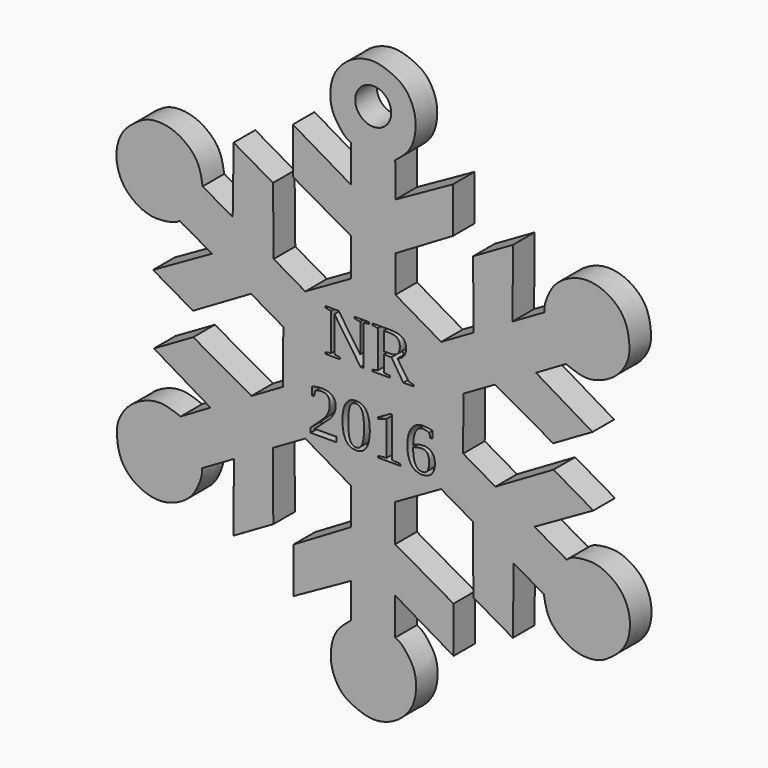
from build123d import *

# Parameters (mm, degrees)
F1_DEPTH     = 3
F3_D         = 4
F4_TEXT_SIZE = 7.1690029775
F5_DEPTH     = 1.5


# Not quite as in the source:
# - Text() gives the source's letters only with a copy of the font that has no kerning and outlines rounded to 1/6400 em; it was checked with that copy


with BuildPart() as f1:
    # F0 (on Front) → F1 (new body)
    with BuildSketch(Plane.XZ):
        with BuildLine():
            add(Edge.make_bspline(
                [(37.2373796999, 9.4348983839), (37.4251641018, 9.3510028964), (37.8701899406, 9.1521809532), (38.6817217589, 8.1752111907), (39.4062988326, 7.0113605624), (39.6519953422, 5.3867909556), (39.3224060532, 3.2517367706), (37.6206347845, 1.2780817822), (35.0148704912, 0.371790515), (32.7778145975, 1.1156204474), (31.2129824114, 1.9875750422), (30.1474541561, 3.8790702997), (29.9862610461, 5.8902465417), (30.532836937, 8.0610699246), (31.7339680071, 9.036908188), (32.3466956615, 9.5347082242)],
                knots=[0, 0, 0, 0, 0.0459998317, 0.1090139196, 0.1754280111, 0.246904677, 0.3288017158, 0.4185892321, 0.5104257569, 0.5955487448, 0.6705198642, 0.7515537915, 0.8317987285, 0.9141962329, 1, 1, 1, 1], degree=3))
            Line((37.2373796999, 9.4348983839), (37.2373796999, 13.5579572657))
            Line((37.2373796999, 13.5579572657), (43.718758629, 9.7468400041))
            Line((43.718758629, 9.7468400041), (43.718758629, 14.8636193613))
            Line((43.718758629, 14.8636193613), (37.2373796999, 18.5688713232))
            Line((37.2373796999, 18.5688713232), (37.2373796999, 22.7115825247))
            Line((37.2373796999, 22.7115825247), (42.3384769651, 25.6261969935))
            Line((42.3384769651, 25.6261969935), (45.8529271634, 23.5971282255))
            Line((45.8529271634, 23.5971282255), (45.9293157475, 16.177781961))
            Line((45.9293157475, 16.177781961), (50.2994563725, 13.6546800947))
            Line((50.2994563725, 13.6546800947), (50.40642864, 20.9681629222))
            Line((50.40642864, 20.9681629222), (53.7508636268, 19.0672780077))
            add(Edge.make_bspline(
                [(56.2826435033, 23.2528297066), (56.4533267724, 23.3765045131), (56.839458541, 23.7361558524), (58.1039257682, 23.9168971573), (59.4727716087, 23.9733834526), (61.002950547, 23.3705901097), (62.6870351656, 22.0186766462), (63.5454277802, 19.5577567309), (63.0273958428, 16.8480186494), (61.264728006, 15.2826441221), (59.7270664918, 14.363176773), (57.556649242, 14.3871852923), (55.7326931115, 15.2492433393), (54.1380932906, 16.8175392077), (53.8742690919, 18.2961027509), (53.7508636268, 19.0672780077)],
                knots=[0, 0, 0, 0, 0.0471420247, 0.110140019, 0.1765371486, 0.2479955595, 0.329871682, 0.4196362669, 0.5114493369, 0.5965505847, 0.6715025566, 0.7525157881, 0.8327402308, 0.9151166911, 1, 1, 1, 1], degree=3))
            Line((56.2826435033, 23.2528297066), (52.7119697703, 25.3143591476))
            Line((52.7119697703, 25.3143591476), (59.2531836002, 29.0218393209))
            Line((59.2531836002, 29.0218393209), (54.8219226914, 31.5802289995))
            Line((54.8219226914, 31.5802289995), (48.3723909003, 27.8198161763))
            Line((48.3723909003, 27.8198161763), (44.7846977593, 29.891171777))
            Line((44.7846977593, 29.891171777), (44.8111162197, 35.7661588302))
            Line((44.8111162197, 35.7661588302), (48.325566418, 37.7952275983))
            Line((48.325566418, 37.7952275983), (54.7891030546, 34.1517089204))
            Line((54.7891030546, 34.1517089204), (59.1592436796, 36.6748107867))
            Line((59.1592436796, 36.6748107867), (52.8790678946, 40.4241929016))
            Line((52.8790678946, 40.4241929016), (56.1975000137, 42.3701161042))
            add(Edge.make_bspline(
                [(53.8385958517, 46.6554776435), (53.8178644494, 46.8551850525), (53.7788826284, 47.3092452721), (54.2124163427, 48.5077384287), (54.8592955807, 49.7124607744), (56.1429910302, 50.7389428582), (58.1569163578, 51.5205869261), (60.7170003528, 51.0337692557), (62.8047652541, 49.2302436061), (63.2791107249, 46.920905952), (63.3064071223, 45.1300249509), (62.2010312841, 43.2603978107), (60.5401138614, 42.1194060959), (58.3836859108, 41.4904279159), (56.9379088943, 42.0872561597), (56.1975000137, 42.3701161042)],
                knots=[0, 0, 0, 0, 0.0449055887, 0.1079742905, 0.1744459427, 0.2459845569, 0.3279525753, 0.4178179099, 0.5097340288, 0.5949307923, 0.6699668886, 0.7510710474, 0.8313855322, 0.91385445, 1, 1, 1, 1], degree=3))
            Line((53.8385958517, 46.6554776435), (50.2679221188, 44.5939482026))
            Line((50.2679221188, 44.5939482026), (50.3277570196, 52.1125456375))
            Line((50.3277570196, 52.1125456375), (45.8964961107, 49.5541559589))
            Line((45.8964961107, 49.5541559589), (45.9283432488, 42.0884911738))
            Line((45.9283432488, 42.0884911738), (42.3406501078, 40.0171355731))
            Line((42.3406501078, 40.0171355731), (37.265971303, 42.9775081575))
            Line((37.265971303, 42.9775081575), (37.265971303, 47.0356456935))
            Line((37.265971303, 47.0356456935), (43.6531193554, 50.8114732802))
            Line((43.6531193554, 50.8114732802), (43.6531193554, 55.8576770127))
            Line((43.6531193554, 55.8576770127), (37.265971303, 52.2935763001))
            Line((37.265971303, 52.2935763001), (37.2399684352, 56.1403844172))
            add(Edge.make_bspline(
                [(32.3492843968, 56.2401942576), (32.1614999949, 56.3240897451), (31.7164741562, 56.5229116883), (30.9049423379, 57.4998814507), (30.1803652642, 58.6637320791), (29.9346687546, 60.2883016859), (30.2642580436, 62.4233558709), (31.9660293123, 64.3970108593), (34.5717936056, 65.3033021265), (36.8088494992, 64.5594721941), (38.3736816853, 63.6875175993), (39.4392099407, 61.7960223418), (39.6004030507, 59.7848460998), (39.0538271598, 57.6140227169), (37.8526960896, 56.6381844535), (37.2399684352, 56.1403844172)],
                knots=[0, 0, 0, 0, 0.0459998317, 0.1090139196, 0.1754280111, 0.246904677, 0.3288017158, 0.4185892321, 0.5104257569, 0.5955487448, 0.6705198642, 0.7515537915, 0.8317987285, 0.9141962329, 1, 1, 1, 1], degree=3))
            Line((32.3492843968, 56.2401942576), (32.3492843968, 52.1171353757))
            Line((32.3492843968, 52.1171353757), (25.8679054677, 55.9282526374))
            Line((25.8679054677, 55.9282526374), (25.8679054677, 50.8114732802))
            Line((25.8679054677, 50.8114732802), (32.3492843968, 47.1062213182))
            Line((32.3492843968, 47.1062213182), (32.3492843968, 42.9635101168))
            Line((32.3492843968, 42.9635101168), (27.2481871317, 40.048895648))
            Line((27.2481871317, 40.048895648), (23.7337369334, 42.077964416))
            Line((23.7337369334, 42.077964416), (23.6573483493, 49.4973106805))
            Line((23.6573483493, 49.4973106805), (19.2872077243, 52.0204125467))
            Line((19.2872077243, 52.0204125467), (19.1802354567, 44.7069297193))
            Line((19.1802354567, 44.7069297193), (15.83580047, 46.6078146338))
            add(Edge.make_bspline(
                [(13.3040205935, 42.4222629348), (13.1374508396, 42.3015687263), (12.7316317675, 42.0337442948), (11.4853994243, 41.8099865936), (10.1133856971, 41.7673638515), (8.5841616668, 42.3659788837), (6.8997724939, 43.719222138), (6.0414744886, 46.1797408304), (6.5594757811, 48.8895645117), (8.3221656598, 50.4550050369), (9.8597733859, 51.3741662906), (12.0303954247, 51.3513774925), (13.8535761538, 50.4846862596), (15.4584642826, 48.9271860463), (15.7107508503, 47.3892644052), (15.83580047, 46.6078146338)],
                knots=[0, 0, 0, 0, 0.0460058885, 0.1090042617, 0.1754017905, 0.2468606312, 0.3287372461, 0.4185023708, 0.510315993, 0.5954177525, 0.6703701752, 0.7513838938, 0.8316088189, 0.9139857747, 1, 1, 1, 1], degree=3))
            Line((13.3040205935, 42.4222629348), (16.8746943265, 40.3607334939))
            Line((16.8746943265, 40.3607334939), (10.3334804965, 36.6532533206))
            Line((10.3334804965, 36.6532533206), (14.7647414054, 34.094863642))
            Line((14.7647414054, 34.094863642), (21.2142731964, 37.8552764652))
            Line((21.2142731964, 37.8552764652), (24.8019663374, 35.7839208645))
            Line((24.8019663374, 35.7839208645), (24.7755478771, 29.9089338112))
            Line((24.7755478771, 29.9089338112), (21.2610976788, 27.8798650432))
            Line((21.2610976788, 27.8798650432), (14.7975610422, 31.5233837211))
            Line((14.7975610422, 31.5233837211), (10.4274204172, 29.0002818548))
            Line((10.4274204172, 29.0002818548), (16.7075962021, 25.2508997399))
            Line((16.7075962021, 25.2508997399), (13.3891640831, 23.3049765373))
            add(Edge.make_bspline(
                [(15.748068245, 19.019614998), (15.7693153188, 18.8149400807), (15.7896746728, 18.3290667003), (15.3647938648, 17.1380098102), (14.714284555, 15.9284244036), (13.4316831295, 14.9034077397), (11.4174097808, 14.1212983992), (8.8574301016, 14.6082517594), (6.7696455939, 16.4117665054), (6.2952734404, 18.7210169673), (6.2680885279, 20.512218795), (7.3730225411, 22.3805839786), (9.0356176295, 23.5263649956), (11.1860400443, 24.1369190986), (12.6491706837, 23.5876777547), (13.3891640831, 23.3049765373)],
                knots=[0, 0, 0, 0, 0.0460225672, 0.1090137068, 0.1754036118, 0.2468542474, 0.3287214612, 0.4184762789, 0.5102793589, 0.5953713469, 0.6703151634, 0.75131958, 0.8315352936, 0.9139027907, 1, 1, 1, 1], degree=3))
            Line((15.748068245, 19.019614998), (19.318741978, 21.0811444389))
            Line((19.318741978, 21.0811444389), (19.2589070772, 13.562547004))
            Line((19.2589070772, 13.562547004), (23.6901679861, 16.1209366826))
            Line((23.6901679861, 16.1209366826), (23.658320848, 23.5866014677))
            Line((23.658320848, 23.5866014677), (27.246013989, 25.6579570684))
            Line((27.246013989, 25.6579570684), (32.3206927938, 22.697584484))
            Line((32.3206927938, 22.697584484), (32.3206927938, 18.6394469479))
            Line((32.3206927938, 18.6394469479), (25.9335447413, 14.8636193613))
            Line((25.9335447413, 14.8636193613), (25.9335447413, 9.8174156288))
            Line((25.9335447413, 9.8174156288), (32.3206927938, 13.3815163413))
            Line((32.3206927938, 13.3815163413), (32.3466956615, 9.5347082242))
        make_face()
    extrude(amount=F1_DEPTH)

    # F3 (through all)
    with Locations(Plane.XZ.offset(3)):
        with Locations((34.794626416, 60.6052711862)):
            Hole(F3_D / 2)

    # F4 (on face) → F5 (cut)
    with BuildSketch(Plane.XZ.offset(3)):
        with Locations((29.3119462052, 34.6608441323)):
            Text('NR', F4_TEXT_SIZE, font='Tinos', text_align=(TextAlign.LEFT, TextAlign.BOTTOM))
        with Locations((27.5196954608, 26.4164907082)):
            Text('2016', F4_TEXT_SIZE, font='Tinos', text_align=(TextAlign.LEFT, TextAlign.BOTTOM))
    extrude(amount=-F5_DEPTH, mode=Mode.SUBTRACT)


solid = f1.part
